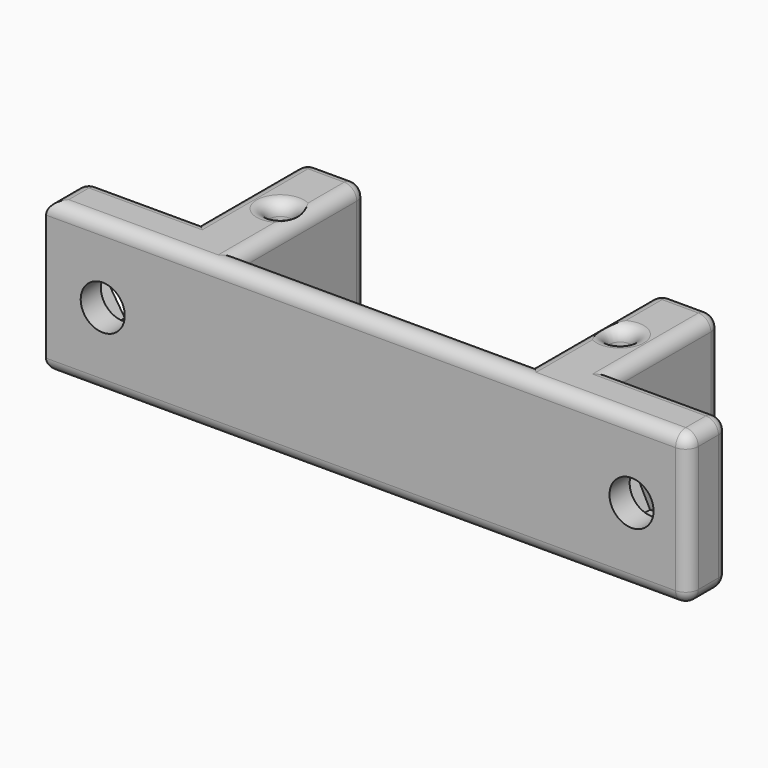
from build123d import *

# Parameters (mm, degrees)
F0_R          = 0.875
F1_DEPTH      = 12
F2_R          = 1.75
F3_DEPTH      = 25
F4_DEPTH      = 2
F5_T1_DEPTH   = 10
F5_T3_DEPTH   = 11.5
F5_T5_DEPTH   = 9.5
F5_T7_DEPTH   = 2.875
F5_T9_DEPTH   = 8
F5_T11_DEPTH  = 5.5
F5_T13_DEPTH  = 52.5
F5_T15_DEPTH  = 2
F5_T17_DEPTH  = 8
F5_T19_DEPTH  = 2.875
F5_T21_DEPTH  = 23.25
F5_S25_W      = 1
F5_S25_H      = 1
F5_T26_DEPTH  = 1
F5_S31_W      = 1
F5_S31_H      = 1
F5_T32_DEPTH  = 1
F5_S37_W      = 1
F5_S37_H      = 1
F5_T38_DEPTH  = 1
F5_S43_W      = 1
F5_S43_H      = 1
F5_T44_DEPTH  = 1
F5_S49_W      = 1
F5_S49_H      = 1
F5_T50_DEPTH  = 1
F5_S55_W      = 1
F5_S55_H      = 1
F5_T56_DEPTH  = 1
F5_S61_W      = 1
F5_S61_H      = 1
F5_T62_DEPTH  = 1
F5_S67_W      = 1
F5_S67_H      = 1
F5_T68_DEPTH  = 1
F5_S73_W      = 1
F5_S73_H      = 1
F5_T74_DEPTH  = 1
F5_S79_W      = 1
F5_S79_H      = 1
F5_T80_DEPTH  = 1
F5_S85_W      = 1
F5_S85_H      = 1
F5_T86_DEPTH  = 1
F5_S91_W      = 1
F5_S91_H      = 1
F5_T92_DEPTH  = 1
F5_S97_W      = 1
F5_S97_H      = 1
F5_T98_DEPTH  = 1
F5_S103_W     = 1
F5_S103_H     = 1
F5_T104_DEPTH = 1
F5_T119_DEPTH = 14
F5_T123_DEPTH = 25.75
F5_T130_DEPTH = 10.5
F5_T134_DEPTH = 12
F5_T141_DEPTH = 12
F5_T145_DEPTH = 10.5
F5_T152_DEPTH = 14
F5_T156_DEPTH = 25.75
F5_T163_DEPTH = 12
F5_T167_DEPTH = 10.5
F5_T174_DEPTH = 10.5
F5_T178_DEPTH = 12
F5_T185_DEPTH = 14
F5_T189_DEPTH = 25.75
F5_T196_DEPTH = 14
F5_T200_DEPTH = 25.75


# Not quite as in the source:
# - a fillet or chamfer that OpenCascade refuses, or shapes differently, is made with other operations: its cross-section is extruded or revolved along the edge and cut away or added


with BuildPart() as f1:
    # F0 (on Top) → F1 (new body)
    with BuildSketch(Plane.XY):
        Polygon((-11.625, 7.25), (-16.5, 7.25), (-16.5, -3.25), (-16.5, -5.25), (-11.625, -5.25), align=None)
        with Locations((-13.5, 1)):
            Circle(F0_R, mode=Mode.SUBTRACT)
        Polygon((11.625, -5.25), (-11.625, -5.25), (-16.5, -5.25), (-16.5, -7.25), (16.5, -7.25), (16.5, -5.25), align=None)
        Polygon((25.5, -3.25), (16.5, -3.25), (16.5, -5.25), (16.5, -7.25), (25.5, -7.25), align=None)
        Polygon((16.5, 7.25), (11.625, 7.25), (11.625, -5.25), (16.5, -5.25), (16.5, -3.25), align=None)
        with Locations((13.5, 1)):
            Circle(F0_R, mode=Mode.SUBTRACT)
        Polygon((-16.5, -5.25), (-16.5, -3.25), (-25.5, -3.25), (-25.5, -7.25), (-16.5, -7.25), align=None)
    extrude(amount=F1_DEPTH)

    # F2 (on face) → F3 (cut)
    with BuildSketch(Plane(origin=(0, -3.25, 0), x_dir=(-1, 0, 0), z_dir=(0, 1, 0))):
        with Locations((-21, 6)):
            Circle(F2_R)
        with Locations((21, 6)):
            Circle(F2_R)
    extrude(amount=-F3_DEPTH, mode=Mode.SUBTRACT)

    # F2 (on face) → F4 (cut)
    with BuildSketch(Plane(origin=(0, -3.25, 0), x_dir=(-1, 0, 0), z_dir=(0, 1, 0))):
        Polygon((19.5559274899, 8.8280714133), (17.8287820573, 6.163432228), (19.2728545674, 3.3353608147), (22.4440725101, 3.1719285867), (24.1712179427, 5.836567772), (22.7271454326, 8.6646391853), align=None)
        with Locations((21, 6)):
            Circle(F2_R, mode=Mode.SUBTRACT)
        Polygon((-22.7271454326, 8.6646391853), (-24.1712179427, 5.836567772), (-22.4440725101, 3.1719285867), (-19.2728545674, 3.3353608147), (-17.8287820573, 6.163432228), (-19.5559274899, 8.8280714133), align=None)
        with Locations((-21, 6)):
            Circle(F2_R, mode=Mode.SUBTRACT)
    extrude(amount=-F4_DEPTH, mode=Mode.SUBTRACT)

    # F5: fillet of radius 1 on 35 edges, made by hand

    # F5_s2 → F5_t1 (cut)
    with BuildSketch(Plane.XY.offset(1)):
        with BuildLine():
            ThreePointArc((16.5, 6.25), (16.2071067812, 6.9571067812), (15.5, 7.25))
            Line((15.5, 7.25), (16.5, 7.25))
            Line((16.5, 7.25), (16.5, 6.25))
        make_face()
        with BuildLine():
            ThreePointArc((12.625, 7.25), (11.9178932188, 6.9571067812), (11.625, 6.25))
            Line((11.625, 6.25), (11.625, 7.25))
            Line((11.625, 7.25), (12.625, 7.25))
        make_face()
        with BuildLine():
            ThreePointArc((-12.625, 7.25), (-11.9178932188, 6.9571067812), (-11.625, 6.25))
            Line((-11.625, 6.25), (-11.625, 7.25))
            Line((-11.625, 7.25), (-12.625, 7.25))
        make_face()
        with BuildLine():
            ThreePointArc((-15.5, 7.25), (-16.2071067812, 6.9571067812), (-16.5, 6.25))
            Line((-16.5, 6.25), (-16.5, 7.25))
            Line((-16.5, 7.25), (-15.5, 7.25))
        make_face()
        with BuildLine():
            ThreePointArc((24.5, -7.25), (25.2071067812, -6.9571067812), (25.5, -6.25))
            Line((25.5, -6.25), (25.5, -7.25))
            Line((25.5, -7.25), (24.5, -7.25))
        make_face()
        with BuildLine():
            ThreePointArc((25.5, -4.25), (25.2071067812, -3.5428932188), (24.5, -3.25))
            Line((24.5, -3.25), (25.5, -3.25))
            Line((25.5, -3.25), (25.5, -4.25))
        make_face()
        with BuildLine():
            ThreePointArc((-24.5, -3.25), (-25.2071067812, -3.5428932188), (-25.5, -4.25))
            Line((-25.5, -4.25), (-25.5, -3.25))
            Line((-25.5, -3.25), (-24.5, -3.25))
        make_face()
    extrude(amount=F5_T1_DEPTH, mode=Mode.SUBTRACT)

    # F5_s4 → F5_t3 (cut)
    with BuildSketch(Plane.XZ.offset(-6.25)):
        with BuildLine():
            ThreePointArc((12.625, 0), (11.9178932188, 0.2928932188), (11.625, 1))
            Line((11.625, 1), (11.625, 0))
            Line((11.625, 0), (12.625, 0))
        make_face()
        with BuildLine():
            ThreePointArc((-11.625, 1), (-11.9178932188, 0.2928932188), (-12.625, 0))
            Line((-12.625, 0), (-11.625, 0))
            Line((-11.625, 0), (-11.625, 1))
        make_face()
        with BuildLine():
            ThreePointArc((12.625, 12), (11.9178932188, 11.7071067812), (11.625, 11))
            Line((11.625, 11), (11.625, 12))
            Line((11.625, 12), (12.625, 12))
        make_face()
        with BuildLine():
            ThreePointArc((-11.625, 11), (-11.9178932188, 11.7071067812), (-12.625, 12))
            Line((-12.625, 12), (-11.625, 12))
            Line((-11.625, 12), (-11.625, 11))
        make_face()
    extrude(amount=F5_T3_DEPTH, mode=Mode.SUBTRACT)

    # F5_s6 → F5_t5 (cut)
    with BuildSketch(Plane.XZ.offset(-6.25)):
        with BuildLine():
            ThreePointArc((15.5, 0), (16.2071067812, 0.2928932188), (16.5, 1))
            Line((16.5, 1), (16.5, 0))
            Line((16.5, 0), (15.5, 0))
        make_face()
        with BuildLine():
            ThreePointArc((-16.5, 1), (-16.2071067812, 0.2928932188), (-15.5, 0))
            Line((-15.5, 0), (-16.5, 0))
            Line((-16.5, 0), (-16.5, 1))
        make_face()
        with BuildLine():
            ThreePointArc((-16.5, 11), (-16.2071067812, 11.7071067812), (-15.5, 12))
            Line((-15.5, 12), (-16.5, 12))
            Line((-16.5, 12), (-16.5, 11))
        make_face()
        with BuildLine():
            ThreePointArc((15.5, 12), (16.2071067812, 11.7071067812), (16.5, 11))
            Line((16.5, 11), (16.5, 12))
            Line((16.5, 12), (15.5, 12))
        make_face()
    extrude(amount=F5_T5_DEPTH, mode=Mode.SUBTRACT)

    # F5_s8 → F5_t7 (cut)
    with BuildSketch(Plane.YZ.offset(-15.5)):
        with BuildLine():
            ThreePointArc((7.25, 1), (6.9571067812, 0.2928932188), (6.25, 0))
            Line((6.25, 0), (7.25, 0))
            Line((7.25, 0), (7.25, 1))
        make_face()
        with BuildLine():
            ThreePointArc((7.25, 11), (6.9571067812, 11.7071067812), (6.25, 12))
            Line((6.25, 12), (7.25, 12))
            Line((7.25, 12), (7.25, 11))
        make_face()
    extrude(amount=F5_T7_DEPTH, mode=Mode.SUBTRACT)

    # F5_s10 → F5_t9 (cut)
    with BuildSketch(Plane.YZ.offset(-24.5)):
        with BuildLine():
            ThreePointArc((-4.25, 0), (-3.5428932188, 0.2928932188), (-3.25, 1))
            Line((-3.25, 1), (-3.25, 0))
            Line((-3.25, 0), (-4.25, 0))
        make_face()
        with BuildLine():
            ThreePointArc((-4.25, 12), (-3.5428932188, 11.7071067812), (-3.25, 11))
            Line((-3.25, 11), (-3.25, 12))
            Line((-3.25, 12), (-4.25, 12))
        make_face()
    extrude(amount=F5_T9_DEPTH, mode=Mode.SUBTRACT)

    # F5_s12 → F5_t11 (cut)
    with BuildSketch(Plane.XZ.offset(4.25)):
        with BuildLine():
            ThreePointArc((-24.5, 0), (-25.2071067812, 0.2928932188), (-25.5, 1))
            Line((-25.5, 1), (-25.5, 0))
            Line((-25.5, 0), (-24.5, 0))
        make_face()
        with BuildLine():
            ThreePointArc((-24.5, 12), (-25.2071067812, 11.7071067812), (-25.5, 11))
            Line((-25.5, 11), (-25.5, 12))
            Line((-25.5, 12), (-24.5, 12))
        make_face()
    extrude(amount=F5_T11_DEPTH, mode=Mode.SUBTRACT)

    # F5_s14 → F5_t13 (cut)
    with BuildSketch(Plane.YZ.offset(-28)):
        with BuildLine():
            ThreePointArc((-6.25, 0), (-6.9571067812, 0.2928932188), (-7.25, 1))
            Line((-7.25, 1), (-7.25, 0))
            Line((-7.25, 0), (-6.25, 0))
        make_face()
        with BuildLine():
            ThreePointArc((-6.25, 12), (-6.9571067812, 11.7071067812), (-7.25, 11))
            Line((-7.25, 11), (-7.25, 12))
            Line((-7.25, 12), (-6.25, 12))
        make_face()
    extrude(amount=F5_T13_DEPTH, mode=Mode.SUBTRACT)

    # F5_s16 → F5_t15 (cut)
    with BuildSketch(Plane.XZ.offset(4.25)):
        with BuildLine():
            ThreePointArc((24.5, 0), (25.2071067812, 0.2928932188), (25.5, 1))
            Line((25.5, 1), (25.5, 0))
            Line((25.5, 0), (24.5, 0))
        make_face()
        with BuildLine():
            ThreePointArc((24.5, 12), (25.2071067812, 11.7071067812), (25.5, 11))
            Line((25.5, 11), (25.5, 12))
            Line((25.5, 12), (24.5, 12))
        make_face()
    extrude(amount=F5_T15_DEPTH, mode=Mode.SUBTRACT)

    # F5_s18 → F5_t17 (cut)
    with BuildSketch(Plane.YZ.offset(16.5)):
        with BuildLine():
            ThreePointArc((-4.25, 0), (-3.5428932188, 0.2928932188), (-3.25, 1))
            Line((-3.25, 1), (-3.25, 0))
            Line((-3.25, 0), (-4.25, 0))
        make_face()
        with BuildLine():
            ThreePointArc((-4.25, 12), (-3.5428932188, 11.7071067812), (-3.25, 11))
            Line((-3.25, 11), (-3.25, 12))
            Line((-3.25, 12), (-4.25, 12))
        make_face()
    extrude(amount=F5_T17_DEPTH, mode=Mode.SUBTRACT)

    # F5_s20 → F5_t19 (cut)
    with BuildSketch(Plane.YZ.offset(12.625)):
        with BuildLine():
            ThreePointArc((6.25, 0), (6.9571067812, 0.2928932188), (7.25, 1))
            Line((7.25, 1), (7.25, 0))
            Line((7.25, 0), (6.25, 0))
        make_face()
        with BuildLine():
            ThreePointArc((6.25, 12), (6.9571067812, 11.7071067812), (7.25, 11))
            Line((7.25, 11), (7.25, 12))
            Line((7.25, 12), (6.25, 12))
        make_face()
    extrude(amount=F5_T19_DEPTH, mode=Mode.SUBTRACT)

    # F5_s22 → F5_t21 (cut)
    with BuildSketch(Plane.YZ.offset(-11.625)):
        with BuildLine():
            ThreePointArc((-6.25, 0), (-5.5428932188, 0.2928932188), (-5.25, 1))
            Line((-5.25, 1), (-5.25, 0))
            Line((-5.25, 0), (-6.25, 0))
        make_face()
        with BuildLine():
            ThreePointArc((-6.25, 12), (-5.5428932188, 11.7071067812), (-5.25, 11))
            Line((-5.25, 11), (-5.25, 12))
            Line((-5.25, 12), (-6.25, 12))
        make_face()
    extrude(amount=F5_T21_DEPTH, mode=Mode.SUBTRACT)


with BuildPart() as f5_tool24:
    # F5_s25 → F5_t26 (new body)
    with BuildSketch(Plane.XY.offset(1)):
        with Locations((16, 6.75)):
            Rectangle(F5_S25_W, F5_S25_H)
    extrude(amount=-F5_T26_DEPTH)

    # F5_s27 → F5_t28 (revolve, cut)
    with BuildSketch(Plane(origin=(15.5, 6.25, 1), x_dir=(-0.7071067812, -0.7071067812, 0), z_dir=(0.7071067812, -0.7071067812, 0))):
        with BuildLine():
            ThreePointArc((0, -1), (1, 0), (0, 1))
            Line((0, 1), (0, -1))
        make_face()
    revolve(axis=Axis((15.5, 6.25, 1), (0, 0, -1)), mode=Mode.SUBTRACT)


with BuildPart() as f1_1:
    add(f1.part)

    # F5_t23: cut F5_tool24
    add(f5_tool24.part, mode=Mode.SUBTRACT)


with BuildPart() as f5_tool30:
    # F5_s31 → F5_t32 (new body)
    with BuildSketch(Plane.YZ.offset(15.5)):
        with Locations((6.75, 11.5)):
            Rectangle(F5_S31_W, F5_S31_H)
    extrude(amount=F5_T32_DEPTH)

    # F5_s33 → F5_t34 (revolve, cut)
    with BuildSketch(Plane(origin=(15.5, 6.25, 11), x_dir=(0, -0.7071067812, -0.7071067812), z_dir=(0, -0.7071067812, 0.7071067812))):
        with BuildLine():
            ThreePointArc((0, -1), (1, 0), (0, 1))
            Line((0, 1), (0, -1))
        make_face()
    revolve(axis=Axis((15.5, 6.25, 11), (1, 0, 0)), mode=Mode.SUBTRACT)


with BuildPart() as f1_2:
    add(f1_1.part)

    # F5_t29: cut F5_tool30
    add(f5_tool30.part, mode=Mode.SUBTRACT)


with BuildPart() as f5_tool36:
    # F5_s37 → F5_t38 (new body)
    with BuildSketch(Plane.XY.offset(1)):
        with Locations((12.125, 6.75)):
            Rectangle(F5_S37_W, F5_S37_H)
    extrude(amount=-F5_T38_DEPTH)

    # F5_s39 → F5_t40 (revolve, cut)
    with BuildSketch(Plane(origin=(12.625, 6.25, 1), x_dir=(0.7071067812, -0.7071067812, 0), z_dir=(0.7071067812, 0.7071067812, 0))):
        with BuildLine():
            ThreePointArc((0, -1), (1, 0), (0, 1))
            Line((0, 1), (0, -1))
        make_face()
    revolve(axis=Axis((12.625, 6.25, 1), (0, 0, -1)), mode=Mode.SUBTRACT)


with BuildPart() as f1_3:
    add(f1_2.part)

    # F5_t35: cut F5_tool36
    add(f5_tool36.part, mode=Mode.SUBTRACT)


with BuildPart() as f5_tool42:
    # F5_s43 → F5_t44 (new body)
    with BuildSketch(Plane.XY.offset(11)):
        with Locations((12.125, 6.75)):
            Rectangle(F5_S43_W, F5_S43_H)
    extrude(amount=F5_T44_DEPTH)

    # F5_s45 → F5_t46 (revolve, cut)
    with BuildSketch(Plane(origin=(12.625, 6.25, 11), x_dir=(0.7071067812, -0.7071067812, 0), z_dir=(-0.7071067812, -0.7071067812, 0))):
        with BuildLine():
            ThreePointArc((0, -1), (1, 0), (0, 1))
            Line((0, 1), (0, -1))
        make_face()
    revolve(axis=Axis((12.625, 6.25, 11), (0, 0, 1)), mode=Mode.SUBTRACT)


with BuildPart() as f1_4:
    add(f1_3.part)

    # F5_t41: cut F5_tool42
    add(f5_tool42.part, mode=Mode.SUBTRACT)


with BuildPart() as f5_tool48:
    # F5_s49 → F5_t50 (new body)
    with BuildSketch(Plane.XZ.offset(-6.25)):
        with Locations((-12.125, 0.5)):
            Rectangle(F5_S49_W, F5_S49_H)
    extrude(amount=-F5_T50_DEPTH)

    # F5_s51 → F5_t52 (revolve, cut)
    with BuildSketch(Plane(origin=(-12.625, 6.25, 1), x_dir=(-0.7071067812, 0, 0.7071067812), z_dir=(-0.7071067812, 0, -0.7071067812))):
        with BuildLine():
            ThreePointArc((0, -1), (1, 0), (0, 1))
            Line((0, 1), (0, -1))
        make_face()
    revolve(axis=Axis((-12.625, 6.25, 1), (0, 1, 0)), mode=Mode.SUBTRACT)


with BuildPart() as f1_5:
    add(f1_4.part)

    # F5_t47: cut F5_tool48
    add(f5_tool48.part, mode=Mode.SUBTRACT)


with BuildPart() as f5_tool54:
    # F5_s55 → F5_t56 (new body)
    with BuildSketch(Plane.XZ.offset(-6.25)):
        with Locations((-12.125, 11.5)):
            Rectangle(F5_S55_W, F5_S55_H)
    extrude(amount=-F5_T56_DEPTH)

    # F5_s57 → F5_t58 (revolve, cut)
    with BuildSketch(Plane(origin=(-12.625, 6.25, 11), x_dir=(-0.7071067812, 0, -0.7071067812), z_dir=(0.7071067812, 0, -0.7071067812))):
        with BuildLine():
            ThreePointArc((0, -1), (1, 0), (0, 1))
            Line((0, 1), (0, -1))
        make_face()
    revolve(axis=Axis((-12.625, 6.25, 11), (0, 1, 0)), mode=Mode.SUBTRACT)


with BuildPart() as f1_6:
    add(f1_5.part)

    # F5_t53: cut F5_tool54
    add(f5_tool54.part, mode=Mode.SUBTRACT)


with BuildPart() as f5_tool60:
    # F5_s61 → F5_t62 (new body)
    with BuildSketch(Plane.XZ.offset(-6.25)):
        with Locations((-16, 0.5)):
            Rectangle(F5_S61_W, F5_S61_H)
    extrude(amount=-F5_T62_DEPTH)

    # F5_s63 → F5_t64 (revolve, cut)
    with BuildSketch(Plane(origin=(-15.5, 6.25, 1), x_dir=(0.7071067812, 0, 0.7071067812), z_dir=(-0.7071067812, 0, 0.7071067812))):
        with BuildLine():
            ThreePointArc((0, -1), (1, 0), (0, 1))
            Line((0, 1), (0, -1))
        make_face()
    revolve(axis=Axis((-15.5, 6.25, 1), (0, 1, 0)), mode=Mode.SUBTRACT)


with BuildPart() as f1_7:
    add(f1_6.part)

    # F5_t59: cut F5_tool60
    add(f5_tool60.part, mode=Mode.SUBTRACT)


with BuildPart() as f5_tool66:
    # F5_s67 → F5_t68 (new body)
    with BuildSketch(Plane.XZ.offset(-6.25)):
        with Locations((-16, 11.5)):
            Rectangle(F5_S67_W, F5_S67_H)
    extrude(amount=-F5_T68_DEPTH)

    # F5_s69 → F5_t70 (revolve, cut)
    with BuildSketch(Plane(origin=(-15.5, 6.25, 11), x_dir=(0.7071067812, 0, -0.7071067812), z_dir=(0.7071067812, 0, 0.7071067812))):
        with BuildLine():
            ThreePointArc((0, -1), (1, 0), (0, 1))
            Line((0, 1), (0, -1))
        make_face()
    revolve(axis=Axis((-15.5, 6.25, 11), (0, 1, 0)), mode=Mode.SUBTRACT)


with BuildPart() as f1_8:
    add(f1_7.part)

    # F5_t65: cut F5_tool66
    add(f5_tool66.part, mode=Mode.SUBTRACT)


with BuildPart() as f5_tool72:
    # F5_s73 → F5_t74 (new body)
    with BuildSketch(Plane.XY.offset(1)):
        with Locations((-25, -3.75)):
            Rectangle(F5_S73_W, F5_S73_H)
    extrude(amount=-F5_T74_DEPTH)

    # F5_s75 → F5_t76 (revolve, cut)
    with BuildSketch(Plane(origin=(-24.5, -4.25, 1), x_dir=(0.7071067812, -0.7071067812, 0), z_dir=(0.7071067812, 0.7071067812, 0))):
        with BuildLine():
            ThreePointArc((0, -1), (1, 0), (0, 1))
            Line((0, 1), (0, -1))
        make_face()
    revolve(axis=Axis((-24.5, -4.25, 1), (0, 0, -1)), mode=Mode.SUBTRACT)


with BuildPart() as f1_9:
    add(f1_8.part)

    # F5_t71: cut F5_tool72
    add(f5_tool72.part, mode=Mode.SUBTRACT)


with BuildPart() as f5_tool78:
    # F5_s79 → F5_t80 (new body)
    with BuildSketch(Plane.XZ.offset(6.25)):
        with Locations((25, 0.5)):
            Rectangle(F5_S79_W, F5_S79_H)
    extrude(amount=F5_T80_DEPTH)

    # F5_s81 → F5_t82 (revolve, cut)
    with BuildSketch(Plane(origin=(24.5, -6.25, 1), x_dir=(-0.7071067812, 0, 0.7071067812), z_dir=(0.7071067812, 0, 0.7071067812))):
        with BuildLine():
            ThreePointArc((0, -1), (1, 0), (0, 1))
            Line((0, 1), (0, -1))
        make_face()
    revolve(axis=Axis((24.5, -6.25, 1), (0, -1, 0)), mode=Mode.SUBTRACT)


with BuildPart() as f1_10:
    add(f1_9.part)

    # F5_t77: cut F5_tool78
    add(f5_tool78.part, mode=Mode.SUBTRACT)


with BuildPart() as f5_tool84:
    # F5_s85 → F5_t86 (new body)
    with BuildSketch(Plane.YZ.offset(24.5)):
        with Locations((-3.75, 0.5)):
            Rectangle(F5_S85_W, F5_S85_H)
    extrude(amount=F5_T86_DEPTH)

    # F5_s87 → F5_t88 (revolve, cut)
    with BuildSketch(Plane(origin=(24.5, -4.25, 1), x_dir=(0, -0.7071067812, 0.7071067812), z_dir=(0, 0.7071067812, 0.7071067812))):
        with BuildLine():
            ThreePointArc((0, -1), (1, 0), (0, 1))
            Line((0, 1), (0, -1))
        make_face()
    revolve(axis=Axis((24.5, -4.25, 1), (1, 0, 0)), mode=Mode.SUBTRACT)


with BuildPart() as f1_11:
    add(f1_10.part)

    # F5_t83: cut F5_tool84
    add(f5_tool84.part, mode=Mode.SUBTRACT)


with BuildPart() as f5_tool90:
    # F5_s91 → F5_t92 (new body)
    with BuildSketch(Plane.XZ.offset(6.25)):
        with Locations((25, 11.5)):
            Rectangle(F5_S91_W, F5_S91_H)
    extrude(amount=F5_T92_DEPTH)

    # F5_s93 → F5_t94 (revolve, cut)
    with BuildSketch(Plane(origin=(24.5, -6.25, 11), x_dir=(-0.7071067812, 0, -0.7071067812), z_dir=(-0.7071067812, 0, 0.7071067812))):
        with BuildLine():
            ThreePointArc((0, -1), (1, 0), (0, 1))
            Line((0, 1), (0, -1))
        make_face()
    revolve(axis=Axis((24.5, -6.25, 11), (0, -1, 0)), mode=Mode.SUBTRACT)


with BuildPart() as f1_12:
    add(f1_11.part)

    # F5_t89: cut F5_tool90
    add(f5_tool90.part, mode=Mode.SUBTRACT)


with BuildPart() as f5_tool96:
    # F5_s97 → F5_t98 (new body)
    with BuildSketch(Plane.YZ.offset(24.5)):
        with Locations((-3.75, 11.5)):
            Rectangle(F5_S97_W, F5_S97_H)
    extrude(amount=F5_T98_DEPTH)

    # F5_s99 → F5_t100 (revolve, cut)
    with BuildSketch(Plane(origin=(24.5, -4.25, 11), x_dir=(0, -0.7071067812, -0.7071067812), z_dir=(0, -0.7071067812, 0.7071067812))):
        with BuildLine():
            ThreePointArc((0, -1), (1, 0), (0, 1))
            Line((0, 1), (0, -1))
        make_face()
    revolve(axis=Axis((24.5, -4.25, 11), (1, 0, 0)), mode=Mode.SUBTRACT)


with BuildPart() as f1_13:
    add(f1_12.part)

    # F5_t95: cut F5_tool96
    add(f5_tool96.part, mode=Mode.SUBTRACT)


with BuildPart() as f5_tool102:
    # F5_s103 → F5_t104 (new body)
    with BuildSketch(Plane.XY.offset(11)):
        with Locations((-25, -3.75)):
            Rectangle(F5_S103_W, F5_S103_H)
    extrude(amount=F5_T104_DEPTH)

    # F5_s105 → F5_t106 (revolve, cut)
    with BuildSketch(Plane(origin=(-24.5, -4.25, 11), x_dir=(0.7071067812, -0.7071067812, 0), z_dir=(-0.7071067812, -0.7071067812, 0))):
        with BuildLine():
            ThreePointArc((0, -1), (1, 0), (0, 1))
            Line((0, 1), (0, -1))
        make_face()
    revolve(axis=Axis((-24.5, -4.25, 11), (0, 0, 1)), mode=Mode.SUBTRACT)


with BuildPart() as f1_14:
    add(f1_13.part)

    # F5_t101: cut F5_tool102
    add(f5_tool102.part, mode=Mode.SUBTRACT)

    # F5_s107 → F5_t108 (revolve, cut)
    with BuildSketch(Plane.XZ.offset(-1)):
        with BuildLine():
            ThreePointArc((-11.625, 0), (-12.3321067812, 0.2928932188), (-12.625, 1))
            Line((-12.625, 1), (-12.625, 0))
            Line((-12.625, 0), (-11.625, 0))
        make_face()
    revolve(axis=Axis((-13.5, 1, 0), (0, 0, 1)), mode=Mode.SUBTRACT)

    # F5_s109 → F5_t110 (revolve, cut)
    with BuildSketch(Plane.XZ.offset(-1)):
        with BuildLine():
            ThreePointArc((15.375, 0), (14.6678932188, 0.2928932188), (14.375, 1))
            Line((14.375, 1), (14.375, 0))
            Line((14.375, 0), (15.375, 0))
        make_face()
    revolve(axis=Axis((13.5, 1, 0), (0, 0, 1)), mode=Mode.SUBTRACT)

    # F5_s111 → F5_t112 (revolve, cut)
    with BuildSketch(Plane.XZ.offset(-1)):
        with BuildLine():
            ThreePointArc((-11.625, 12), (-12.3321067812, 11.7071067812), (-12.625, 11))
            Line((-12.625, 11), (-12.625, 12))
            Line((-12.625, 12), (-11.625, 12))
        make_face()
    revolve(axis=Axis((-13.5, 1, 12), (0, 0, 1)), mode=Mode.SUBTRACT)

    # F5_s113 → F5_t114 (revolve, cut)
    with BuildSketch(Plane.XZ.offset(-1)):
        with BuildLine():
            ThreePointArc((15.375, 12), (14.6678932188, 11.7071067812), (14.375, 11))
            Line((14.375, 11), (14.375, 12))
            Line((14.375, 12), (15.375, 12))
        make_face()
    revolve(axis=Axis((13.5, 1, 12), (0, 0, 1)), mode=Mode.SUBTRACT)


with BuildPart() as f5_tool117:
    # F5_s118 → F5_t119 (new body)
    with BuildSketch(Plane.XZ.offset(-6.25)):
        with BuildLine():
            ThreePointArc((12.625, 0), (11.9178932188, 0.2928932188), (11.625, 1))
            Line((11.625, 1), (11.625, 0))
            Line((11.625, 0), (12.625, 0))
        make_face()
    extrude(amount=F5_T119_DEPTH)

    split(bisect_by=Plane.XZ.offset(5.25), keep=Keep.TOP)


with BuildPart() as f5_tool121:
    # F5_s122 → F5_t123 (new body)
    with BuildSketch(Plane.YZ.offset(14.125)):
        with BuildLine():
            ThreePointArc((-6.25, 0), (-5.5428932188, 0.2928932188), (-5.25, 1))
            Line((-5.25, 1), (-5.25, 0))
            Line((-5.25, 0), (-6.25, 0))
        make_face()
    extrude(amount=-F5_T123_DEPTH)

    split(bisect_by=Plane.YZ.offset(11.625), keep=Keep.TOP)


with BuildPart() as f5_tool117_1:
    add(f5_tool117.part)

    # F5_t125: intersect F5_tool121
    add(f5_tool121.part, mode=Mode.INTERSECT)


with BuildPart() as f1_15:
    add(f1_14.part)

    # F5_t115: cut F5_tool117
    add(f5_tool117_1.part, mode=Mode.SUBTRACT)


with BuildPart() as f5_tool128:
    # F5_s129 → F5_t130 (new body)
    with BuildSketch(Plane.YZ.offset(24.5)):
        with BuildLine():
            ThreePointArc((-4.25, 0), (-3.5428932188, 0.2928932188), (-3.25, 1))
            Line((-3.25, 1), (-3.25, 0))
            Line((-3.25, 0), (-4.25, 0))
        make_face()
    extrude(amount=-F5_T130_DEPTH)

    split(bisect_by=Plane.YZ.offset(16.5), keep=Keep.BOTTOM)


with BuildPart() as f5_tool132:
    # F5_s133 → F5_t134 (new body)
    with BuildSketch(Plane.XZ.offset(5.75)):
        with BuildLine():
            ThreePointArc((15.5, 0), (16.2071067812, 0.2928932188), (16.5, 1))
            Line((16.5, 1), (16.5, 0))
            Line((16.5, 0), (15.5, 0))
        make_face()
    extrude(amount=-F5_T134_DEPTH)

    split(bisect_by=Plane.XZ.offset(3.25), keep=Keep.TOP)


with BuildPart() as f5_tool128_1:
    add(f5_tool128.part)

    # F5_t136: intersect F5_tool132
    add(f5_tool132.part, mode=Mode.INTERSECT)


with BuildPart() as f1_16:
    add(f1_15.part)

    # F5_t126: cut F5_tool128
    add(f5_tool128_1.part, mode=Mode.SUBTRACT)


with BuildPart() as f5_tool139:
    # F5_s140 → F5_t141 (new body)
    with BuildSketch(Plane.XZ.offset(-6.25)):
        with BuildLine():
            ThreePointArc((-16.5, 1), (-16.2071067812, 0.2928932188), (-15.5, 0))
            Line((-15.5, 0), (-16.5, 0))
            Line((-16.5, 0), (-16.5, 1))
        make_face()
    extrude(amount=F5_T141_DEPTH)

    split(bisect_by=Plane.XZ.offset(3.25), keep=Keep.TOP)


with BuildPart() as f5_tool143:
    # F5_s144 → F5_t145 (new body)
    with BuildSketch(Plane.YZ.offset(-14)):
        with BuildLine():
            ThreePointArc((-4.25, 0), (-3.5428932188, 0.2928932188), (-3.25, 1))
            Line((-3.25, 1), (-3.25, 0))
            Line((-3.25, 0), (-4.25, 0))
        make_face()
    extrude(amount=-F5_T145_DEPTH)

    split(bisect_by=Plane.YZ.offset(-16.5), keep=Keep.TOP)


with BuildPart() as f5_tool139_1:
    add(f5_tool139.part)

    # F5_t147: intersect F5_tool143
    add(f5_tool143.part, mode=Mode.INTERSECT)


with BuildPart() as f1_17:
    add(f1_16.part)

    # F5_t137: cut F5_tool139
    add(f5_tool139_1.part, mode=Mode.SUBTRACT)


with BuildPart() as f5_tool150:
    # F5_s151 → F5_t152 (new body)
    with BuildSketch(Plane.XZ.offset(7.75)):
        with BuildLine():
            ThreePointArc((-11.625, 1), (-11.9178932188, 0.2928932188), (-12.625, 0))
            Line((-12.625, 0), (-11.625, 0))
            Line((-11.625, 0), (-11.625, 1))
        make_face()
    extrude(amount=-F5_T152_DEPTH)

    split(bisect_by=Plane.XZ.offset(5.25), keep=Keep.TOP)


with BuildPart() as f5_tool154:
    # F5_s155 → F5_t156 (new body)
    with BuildSketch(Plane.YZ.offset(11.625)):
        with BuildLine():
            ThreePointArc((-6.25, 0), (-5.5428932188, 0.2928932188), (-5.25, 1))
            Line((-5.25, 1), (-5.25, 0))
            Line((-5.25, 0), (-6.25, 0))
        make_face()
    extrude(amount=-F5_T156_DEPTH)

    split(bisect_by=Plane.YZ.offset(-11.625), keep=Keep.BOTTOM)


with BuildPart() as f5_tool150_1:
    add(f5_tool150.part)

    # F5_t158: intersect F5_tool154
    add(f5_tool154.part, mode=Mode.INTERSECT)


with BuildPart() as f1_18:
    add(f1_17.part)

    # F5_t148: cut F5_tool150
    add(f5_tool150_1.part, mode=Mode.SUBTRACT)


with BuildPart() as f5_tool161:
    # F5_s162 → F5_t163 (new body)
    with BuildSketch(Plane.XZ.offset(-6.25)):
        with BuildLine():
            ThreePointArc((-16.5, 11), (-16.2071067812, 11.7071067812), (-15.5, 12))
            Line((-15.5, 12), (-16.5, 12))
            Line((-16.5, 12), (-16.5, 11))
        make_face()
    extrude(amount=F5_T163_DEPTH)

    split(bisect_by=Plane.XZ.offset(3.25), keep=Keep.TOP)


with BuildPart() as f5_tool165:
    # F5_s166 → F5_t167 (new body)
    with BuildSketch(Plane.YZ.offset(-14)):
        with BuildLine():
            ThreePointArc((-4.25, 12), (-3.5428932188, 11.7071067812), (-3.25, 11))
            Line((-3.25, 11), (-3.25, 12))
            Line((-3.25, 12), (-4.25, 12))
        make_face()
    extrude(amount=-F5_T167_DEPTH)

    split(bisect_by=Plane.YZ.offset(-16.5), keep=Keep.TOP)


with BuildPart() as f5_tool161_1:
    add(f5_tool161.part)

    # F5_t169: intersect F5_tool165
    add(f5_tool165.part, mode=Mode.INTERSECT)


with BuildPart() as f1_19:
    add(f1_18.part)

    # F5_t159: cut F5_tool161
    add(f5_tool161_1.part, mode=Mode.SUBTRACT)


with BuildPart() as f5_tool172:
    # F5_s173 → F5_t174 (new body)
    with BuildSketch(Plane.YZ.offset(24.5)):
        with BuildLine():
            ThreePointArc((-4.25, 12), (-3.5428932188, 11.7071067812), (-3.25, 11))
            Line((-3.25, 11), (-3.25, 12))
            Line((-3.25, 12), (-4.25, 12))
        make_face()
    extrude(amount=-F5_T174_DEPTH)

    split(bisect_by=Plane.YZ.offset(16.5), keep=Keep.BOTTOM)


with BuildPart() as f5_tool176:
    # F5_s177 → F5_t178 (new body)
    with BuildSketch(Plane.XZ.offset(5.75)):
        with BuildLine():
            ThreePointArc((15.5, 12), (16.2071067812, 11.7071067812), (16.5, 11))
            Line((16.5, 11), (16.5, 12))
            Line((16.5, 12), (15.5, 12))
        make_face()
    extrude(amount=-F5_T178_DEPTH)

    split(bisect_by=Plane.XZ.offset(3.25), keep=Keep.TOP)


with BuildPart() as f5_tool172_1:
    add(f5_tool172.part)

    # F5_t180: intersect F5_tool176
    add(f5_tool176.part, mode=Mode.INTERSECT)


with BuildPart() as f1_20:
    add(f1_19.part)

    # F5_t170: cut F5_tool172
    add(f5_tool172_1.part, mode=Mode.SUBTRACT)


with BuildPart() as f5_tool183:
    # F5_s184 → F5_t185 (new body)
    with BuildSketch(Plane.XZ.offset(-6.25)):
        with BuildLine():
            ThreePointArc((12.625, 12), (11.9178932188, 11.7071067812), (11.625, 11))
            Line((11.625, 11), (11.625, 12))
            Line((11.625, 12), (12.625, 12))
        make_face()
    extrude(amount=F5_T185_DEPTH)

    split(bisect_by=Plane.XZ.offset(5.25), keep=Keep.TOP)


with BuildPart() as f5_tool187:
    # F5_s188 → F5_t189 (new body)
    with BuildSketch(Plane.YZ.offset(14.125)):
        with BuildLine():
            ThreePointArc((-6.25, 12), (-5.5428932188, 11.7071067812), (-5.25, 11))
            Line((-5.25, 11), (-5.25, 12))
            Line((-5.25, 12), (-6.25, 12))
        make_face()
    extrude(amount=-F5_T189_DEPTH)

    split(bisect_by=Plane.YZ.offset(11.625), keep=Keep.TOP)


with BuildPart() as f5_tool183_1:
    add(f5_tool183.part)

    # F5_t191: intersect F5_tool187
    add(f5_tool187.part, mode=Mode.INTERSECT)


with BuildPart() as f1_21:
    add(f1_20.part)

    # F5_t181: cut F5_tool183
    add(f5_tool183_1.part, mode=Mode.SUBTRACT)


with BuildPart() as f5_tool194:
    # F5_s195 → F5_t196 (new body)
    with BuildSketch(Plane.XZ.offset(7.75)):
        with BuildLine():
            ThreePointArc((-11.625, 11), (-11.9178932188, 11.7071067812), (-12.625, 12))
            Line((-12.625, 12), (-11.625, 12))
            Line((-11.625, 12), (-11.625, 11))
        make_face()
    extrude(amount=-F5_T196_DEPTH)

    split(bisect_by=Plane.XZ.offset(5.25), keep=Keep.TOP)


with BuildPart() as f5_tool198:
    # F5_s199 → F5_t200 (new body)
    with BuildSketch(Plane.YZ.offset(11.625)):
        with BuildLine():
            ThreePointArc((-6.25, 12), (-5.5428932188, 11.7071067812), (-5.25, 11))
            Line((-5.25, 11), (-5.25, 12))
            Line((-5.25, 12), (-6.25, 12))
        make_face()
    extrude(amount=-F5_T200_DEPTH)

    split(bisect_by=Plane.YZ.offset(-11.625), keep=Keep.BOTTOM)


with BuildPart() as f5_tool194_1:
    add(f5_tool194.part)

    # F5_t202: intersect F5_tool198
    add(f5_tool198.part, mode=Mode.INTERSECT)


with BuildPart() as f1_22:
    add(f1_21.part)

    # F5_t192: cut F5_tool194
    add(f5_tool194_1.part, mode=Mode.SUBTRACT)


solid = f1_22.part
